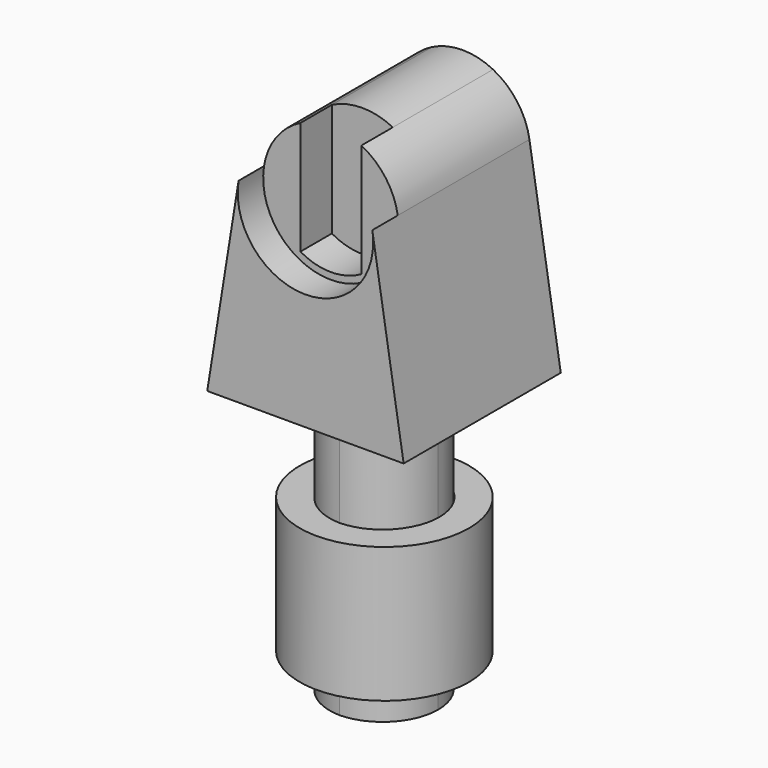
from build123d import *

# Parameters (mm, degrees)
F1_DEPTH    = 29
F2_DEPTH    = 18.5
F3_DEPTH    = 24.3
F4_START    = 6.3
F0_W        = 16
F0_H        = 35
F4_DEPTH    = 16.4
F5_T1_DEPTH = 60.5
F7_START    = -15
F6_R        = 12.5
F6_R_2      = 8.0882914417
F7_DEPTH    = 20


# Not quite as in the source:
# - a fillet or chamfer that OpenCascade refuses, or shapes differently, is made with other operations: its cross-section is extruded or revolved along the edge and cut away or added


with BuildPart() as f1:
    # F0 (on Front) → F1 (new body)
    with BuildSketch(Plane.XZ):
        with BuildLine():
            Line((-8, 0), (0, 0))
            Line((0, 0), (8, 0))
            Line((8, 0), (8.2, 0))
            Line((8.2, 0), (14.5, 0))
            Line((14.5, 0), (9.873721074, 28.8341818559))
            ThreePointArc((9.873721074, 28.8341818559), (9.9683802782, 28.0446034419), (10, 27.25))
            ThreePointArc((10, 27.25), (-0.7946034419, 17.2816197218), (-9.873721074, 28.8341818559))
            Line((-9.873721074, 28.8341818559), (-14.5, 0))
            Line((-14.5, 0), (-8.2, 0))
            Line((-8.2, 0), (-8, 0))
        make_face()
    extrude(amount=F1_DEPTH)



with BuildPart() as f2:
    # F0 (on Front) → F2 (new body)
    with BuildSketch(Plane.XZ):
        with BuildLine():
            Line((4.5, 35.0442286341), (4.5, 36.1802855497))
            ThreePointArc((4.5, 36.1802855497), (0, 37.25), (-4.5, 36.1802855497))
            Line((-4.5, 36.1802855497), (-4.5, 35.0442286341))
            Line((-4.5, 35.0442286341), (-4.5, 19.4557713659))
            ThreePointArc((-4.5, 19.4557713659), (0, 18.25), (4.5, 19.4557713659))
            Line((4.5, 19.4557713659), (4.5, 35.0442286341))
        make_face()
        with BuildLine():
            ThreePointArc((4.5, 19.4557713659), (9, 27.25), (4.5, 35.0442286341))
            Line((4.5, 35.0442286341), (4.5, 19.4557713659))
        make_face()
    extrude(amount=F2_DEPTH)


with BuildPart() as f1_1:
    add(f1.part)

    add(f2.part)  # F3 merges F2
    # F0 (on Front) → F3 (join)
    with BuildSketch(Plane.XZ):
        with BuildLine():
            ThreePointArc((10, 27.25), (9.9683802782, 28.0446034419), (9.873721074, 28.8341818559))
            ThreePointArc((9.873721074, 28.8341818559), (8.0710763996, 33.1540431698), (4.5, 36.1802855497))
            Line((4.5, 36.1802855497), (4.5, 35.0442286341))
            ThreePointArc((4.5, 35.0442286341), (9, 27.25), (4.5, 19.4557713659))
            ThreePointArc((4.5, 19.4557713659), (0, 18.25), (-4.5, 19.4557713659))
            ThreePointArc((-4.5, 19.4557713659), (-9, 27.25), (-4.5, 35.0442286341))
            Line((-4.5, 35.0442286341), (-4.5, 36.1802855497))
            ThreePointArc((-4.5, 36.1802855497), (-8.0710763996, 33.1540431698), (-9.873721074, 28.8341818559))
            ThreePointArc((-9.873721074, 28.8341818559), (-0.7946034419, 17.2816197218), (10, 27.25))
        make_face()
        with BuildLine():
            ThreePointArc((4.5, 19.4557713659), (9, 27.25), (4.5, 35.0442286341))
            Line((4.5, 35.0442286341), (4.5, 19.4557713659))
        make_face()
        with BuildLine():
            Line((-4.5, 19.4557713659), (-4.5, 35.0442286341))
            ThreePointArc((-4.5, 35.0442286341), (-9, 27.25), (-4.5, 19.4557713659))
        make_face()
    extrude(amount=F3_DEPTH)

    # F0 (on Front) → F4 (join)
    with BuildSketch(Plane.XZ.offset(F4_START)):
        with Locations((0, -22.5)):
            Rectangle(F0_W, F0_H)
        Polygon((8, 0), (0, 0), (-8, 0), (-8, -5), (8, -5), align=None)
    extrude(amount=F4_DEPTH)

    # F5: fillet of radius 8.2 on 4 edges, made by hand

    # F5_s2 → F5_t1 (cut)
    with BuildSketch(Plane.XY.offset(-60.5)):
        with BuildLine():
            ThreePointArc((0.2, -6.3), (-5.5982756057, -8.7017243943), (-8, -14.5))
            Line((-8, -14.5), (-8, -6.3))
            Line((-8, -6.3), (0.2, -6.3))
        make_face()
        with BuildLine():
            ThreePointArc((-8, -14.5), (-5.5982756057, -20.2982756057), (0.2, -22.7))
            Line((0.2, -22.7), (-8, -22.7))
            Line((-8, -22.7), (-8, -14.5))
        make_face()
        with BuildLine():
            ThreePointArc((-0.2, -6.3), (5.5982756057, -8.7017243943), (8, -14.5))
            Line((8, -14.5), (8, -6.3))
            Line((8, -6.3), (-0.2, -6.3))
        make_face()
        with BuildLine():
            ThreePointArc((-0.2, -22.7), (5.5982756057, -20.2982756057), (8, -14.5))
            Line((8, -14.5), (8, -22.7))
            Line((8, -22.7), (-0.2, -22.7))
        make_face()
    extrude(amount=F5_T1_DEPTH, mode=Mode.SUBTRACT)


with BuildPart() as f7:
    # F6 (on Top) → F7 (new body)
    with BuildSketch(Plane.XY.offset(F7_START)):
        with Locations((-0.0183524884, -14.4015014629)):
            Circle(F6_R)
        with Locations((-0.0183524884, -14.4015014629)):
            Circle(F6_R_2, mode=Mode.SUBTRACT)
    extrude(amount=-F7_DEPTH)


solid = Compound([f1_1.part, f7.part])
